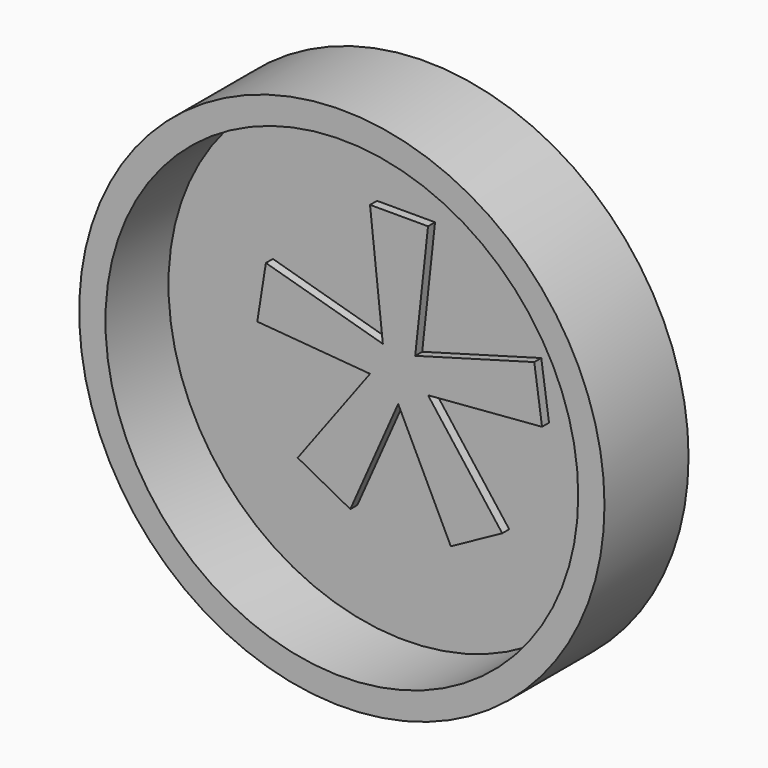
from build123d import *

# Parameters (mm, degrees)
F0_R         = 30
F1_DEPTH     = 12
F2_T         = -3
F3_TEXT_SIZE = 69.964471167
F4_DEPTH     = 1


# Not quite as in the source:
# - Text() gives the source's letters only with a copy of the font that has no kerning and outlines rounded to 1/6400 em; it was checked with that copy


with BuildPart() as f1:
    # F0 (on Front) → F1 (new body)
    with BuildSketch(Plane.XZ):
        Circle(F0_R)
    extrude(amount=F1_DEPTH)

    # F2
    f2_openings = [f1.faces().sort_by_distance(p)[0] for p in [
        (0, -12, 0),
    ]]
    offset(amount=F2_T, openings=f2_openings)

    # F3 (on face) → F4 (join)
    with BuildSketch(Plane.XZ.offset(3)):
        with Locations((-19, -37)):
            Text('*', F3_TEXT_SIZE, font='Open Sans', text_align=(TextAlign.LEFT, TextAlign.BOTTOM))
    extrude(amount=F4_DEPTH)


solid = f1.part
